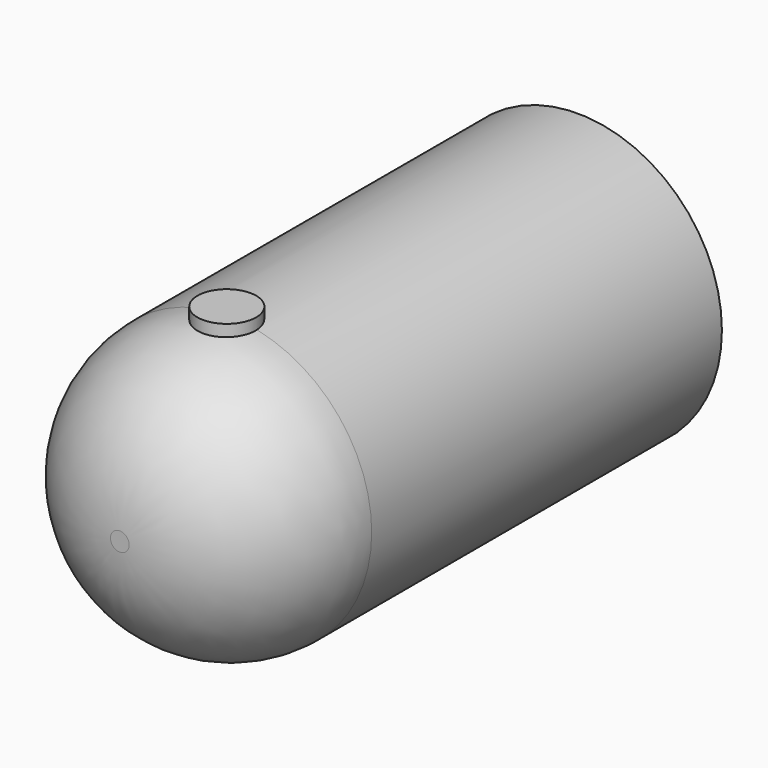
from build123d import *

# Parameters (mm, degrees)
F0_R     = 29.9274598154
F1_DEPTH = 75.92757
F2_R     = 27.9824251374
F3_DEPTH = 42.964930072
F4_R     = 6.0972524399
F5_DEPTH = 31.6609
F6_DEPTH = 6.63492


# Not quite as in the source:
# - a feature names something its author has since deleted; it is built from what else it names


with BuildPart() as f1:
    # F0 (on Front) → F1 (new body)
    with BuildSketch(Plane.XZ):
        Circle(F0_R)
    extrude(amount=F1_DEPTH)

    # F2
    f2_edges = [f1.edges().sort_by_distance(p)[0] for p in [
        (-29.92746, -75.92757, 0),
    ]]
    fillet(f2_edges, radius=F2_R)

    # F3 (add): a face of the model
    f3_faces = [f1.faces().sort_by_distance(p)[0] for p in [
        (0, 0, 0),
    ]]
    extrude(f3_faces, amount=F3_DEPTH)

    # F4 (on Top) → F5 (join)
    with BuildSketch(Plane.XY):
        with Locations((0, -48.1517650187)):
            Circle(F4_R)
    extrude(amount=F5_DEPTH)

    # F6 (add): a face of the model
    f6_faces = [f1.faces().sort_by_distance(p)[0] for p in [
        (0, -48.1517650187, 31.6609),
    ]]
    extrude(f6_faces, amount=-F6_DEPTH)


solid = f1.part
